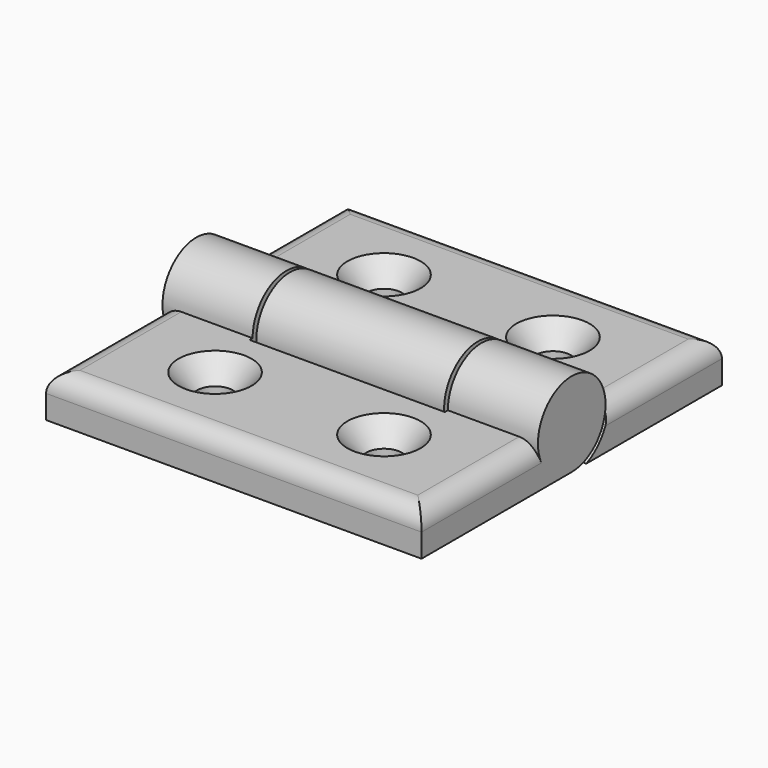
from build123d import *

# Parameters (mm, degrees)
F5_W              = 15.5
F5_H              = 4.5
F8_DEPTH          = 10
F8_DEPTH_BACK     = 10
F9_W              = 0.4
F9_H              = 4.5
F10_DEPTH         = 9.6
F12_DEPTH         = 9.6
F13_DEPTH         = 9.6
F11_W             = 0.4
F11_H             = 4.5
F14_DEPTH         = 9.6
F9_W_2            = 15.1
F15_DEPTH         = 40
F17_DEPTH         = 10
F19_DEPTH         = 10
F20_R             = 2
F20_2_R           = 2
F22_D             = 3.7973
F22_CSINK_D       = 7.7978
F22_CSINK_ANGLE   = 82
F22_2_D           = 3.7973
F22_2_CSINK_D     = 7.7978
F22_2_CSINK_ANGLE = 82


with BuildPart() as f3:
    # F2 (on Front) → F3 (revolve)
    with BuildSketch(Plane.XZ):
        with BuildLine():
            Line((-10, 2.5590475353), (-10, 0))
            Line((-10, 0), (10, 0))
            Line((10, 0), (10, 2.4063855079))
            ThreePointArc((10, 2.4063855079), (-0.0074897347, 1.5014987586), (-10, 2.5590475353))
        make_face()
        with BuildLine():
            Line((-10.4, 0), (-10, 0))
            Line((-10, 0), (-10, 2.5590475353))
            ThreePointArc((-10, 2.5590475353), (-10.2000835145, 2.6006984263), (-10.4, 2.6431437831))
            Line((-10.4, 2.6431437831), (-10.4, 0))
        make_face()
        with BuildLine():
            Line((10, 2.4063855079), (10, 0))
            Line((10, 0), (10.4, 0))
            Line((10.4, 0), (10.4, 2.484120304))
            ThreePointArc((10.4, 2.484120304), (10.2000769588, 2.4448568988), (10, 2.4063855079))
        make_face()
    revolve(axis=Axis((0, 0, 0), (1, 0, 0)))

    # F9 (on offset) → F10 (join, through all)
    with BuildSketch(Plane.YZ.offset(20)):
        with Locations((-4.7, -2.25)):
            Rectangle(F9_W, F9_H)
        with BuildLine():
            ThreePointArc((4.5, 0), (0, 4.5), (-4.5, 0))
            Line((-4.5, 0), (4.5, 0))
        make_face()
        with BuildLine():
            ThreePointArc((0, -4.5), (-3.1819805153, -3.1819805153), (-4.5, 0))
            Line((-4.5, 0), (-4.5, -4.5))
            Line((-4.5, -4.5), (0, -4.5))
        make_face()
        with BuildLine():
            Line((4.5, 0), (-4.5, 0))
            ThreePointArc((-4.5, 0), (-3.1819805153, -3.1819805153), (0, -4.5))
            ThreePointArc((0, -4.5), (3.1819805153, -3.1819805153), (4.5, 0))
        make_face()
    extrude(amount=-F10_DEPTH)

    # F11 (on offset) → F12 (join, through all)
    with BuildSketch(Plane.YZ.offset(-20)):
        with BuildLine():
            ThreePointArc((0, -4.5), (3.1819805153, -3.1819805153), (4.5, 0))
            Line((4.5, 0), (-4.5, 0))
            ThreePointArc((-4.5, 0), (-3.1819805153, -3.1819805153), (0, -4.5))
        make_face()
        with BuildLine():
            Line((-4.5, 0), (4.5, 0))
            ThreePointArc((4.5, 0), (0, 4.5), (-4.5, 0))
        make_face()
        with BuildLine():
            ThreePointArc((0, -4.5), (-3.1819805153, -3.1819805153), (-4.5, 0))
            Line((-4.5, 0), (-4.5, -4.5))
            Line((-4.5, -4.5), (0, -4.5))
        make_face()
    extrude(amount=F12_DEPTH)

    # F9 (on offset) → F13 (join)
    with BuildSketch(Plane.YZ.offset(20)):
        with Locations((-4.7, -2.25)):
            Rectangle(F9_W, F9_H)
    extrude(amount=-F13_DEPTH)

    # F11 (on offset) → F14 (join)
    with BuildSketch(Plane.YZ.offset(-20)):
        with Locations((-4.7, -2.25)):
            Rectangle(F11_W, F11_H)
    extrude(amount=F14_DEPTH)

    # F9 (on offset) → F15 (join, through all)
    with BuildSketch(Plane.YZ.offset(20)):
        with Locations((-12.45, -2.25)):
            Rectangle(F9_W_2, F9_H)
    extrude(amount=-F15_DEPTH)

    # F20
    f20_edges = [f3.edges().sort_by_distance(p)[0] for p in [
        (20, -12.25, 0),
        (0, -20, 0),
        (-20, -12.25, 0),
    ]]
    fillet(f20_edges, radius=F20_R)

    # F22 (through all)
    with Locations(Plane.XY):
        with Locations((9, 11.25), (-9, 11.25), (-9, -11.25), (9, -11.25)):
            CounterSinkHole(F22_D / 2, F22_CSINK_D / 2, counter_sink_angle=F22_CSINK_ANGLE)


with BuildPart() as f4:
    # F2 (on Front) → F4 (revolve)
    with BuildSketch(Plane.XZ):
        with BuildLine():
            Line((-10, 4.5), (-10, 2.9675223036))
            ThreePointArc((-10, 2.9675223036), (-0.0076110898, 1.9015114363), (10, 2.8136164617))
            Line((10, 2.8136164617), (10, 4.5))
            Line((10, 4.5), (-10, 4.5))
        make_face()
    revolve(axis=Axis((0, 0, 0), (1, 0, 0)))

    # F5 (on Right) → F8 (join, two sides)
    with BuildSketch(Plane.YZ) as f8_sk:
        with Locations((12.25, -2.25)):
            Rectangle(F5_W, F5_H)
        with BuildLine():
            Line((4.5, -4.5), (4.5, 0))
            ThreePointArc((4.5, 0), (3.1819805153, -3.1819805153), (0, -4.5))
            Line((0, -4.5), (4.5, -4.5))
        make_face()
    extrude(amount=F8_DEPTH)
    extrude(f8_sk.sketch, amount=-F8_DEPTH_BACK)

    # F16 (on face) → F17 (join, through all)
    with BuildSketch(Plane(origin=(-10, 0, 0), x_dir=(0, -1, 0), z_dir=(-1, 0, 0))):
        with BuildLine():
            ThreePointArc((-1.939071943, -4.5), (-4.0933759002, -2.6933759002), (-4.9, 0))
            Line((-4.9, 0), (-20, 0))
            Line((-20, 0), (-20, -4.5))
            Line((-20, -4.5), (-1.939071943, -4.5))
        make_face()
    extrude(amount=F17_DEPTH)

    # F18 (on face) → F19 (join, through all)
    with BuildSketch(Plane.YZ.offset(10)):
        with BuildLine():
            Line((20, 0), (4.9, 0))
            ThreePointArc((4.9, 0), (4.0933759002, -2.6933759002), (1.939071943, -4.5))
            Line((1.939071943, -4.5), (20, -4.5))
            Line((20, -4.5), (20, 0))
        make_face()
    extrude(amount=F19_DEPTH)

    # F20#2
    f20_2_edges = [f4.edges().sort_by_distance(p)[0] for p in [
        (20, 12.45, 0),
        (0, 20, 0),
        (-20, 12.45, 0),
    ]]
    fillet(f20_2_edges, radius=F20_2_R)

    # F22#2 (through all)
    with Locations(Plane.XY):
        with Locations((9, 11.25), (-9, 11.25), (-9, -11.25), (9, -11.25)):
            CounterSinkHole(F22_2_D / 2, F22_2_CSINK_D / 2, counter_sink_angle=F22_2_CSINK_ANGLE)


solid = Compound([f3.part, f4.part])
